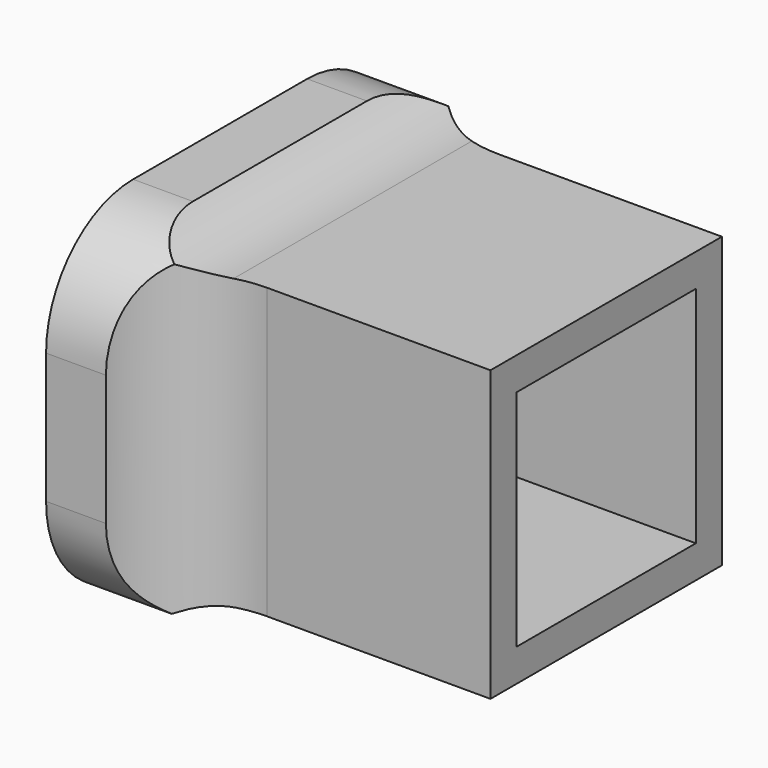
from build123d import *

# Parameters (mm, degrees)
F0_W         = 2.75
F0_H         = 20
F1_DEPTH     = 16
F2_W         = 5.15
F2_H         = 10.3
F3_DEPTH     = 2.75
F4_DEPTH     = 15
F5_T1_DEPTH  = 13.2999992773
F5_T3_DEPTH  = 13.2999992773
F5_T9_DEPTH  = 21.6634917276
F5_T14_DEPTH = 25.0997612432
F5_T22_DEPTH = 21.6634917276
F5_T27_DEPTH = 25.0997612432
F5_T35_DEPTH = 22.0158699277
F5_T40_DEPTH = 25.0997612432
F5_T48_DEPTH = 25.0997612432
F5_T53_DEPTH = 22.0158699277
F6_R         = 5


# Not quite as in the source:
# - a fillet or chamfer that OpenCascade refuses, or shapes differently, is made with other operations: its cross-section is extruded or revolved along the edge and cut away or added
# - a feature names something its author has since deleted; it is built from what else it names


with BuildPart() as f1:
    # F0 (on Top) → F1 (new body)
    with BuildSketch(Plane.XY):
        Rectangle(F0_W, F0_H)
    extrude(amount=F1_DEPTH)

    # F2 (on face) → F3 (join)
    with BuildSketch(Plane.YZ.offset(1.375)):
        Polygon((0, 16), (-10, 16), (-10, 0), (0, 0), (0, 1.4159553841), (-6.6499996386, 1.4159553841), (-6.6499996386, 14.7159546614), (0, 14.7159546614), align=None)
        Polygon((10, 16), (0, 16), (0, 14.7159546614), (6.6499996386, 14.7159546614), (6.6499996386, 1.4159553841), (0, 1.4159553841), (0, 0), (10, 0), align=None)
        with Locations((-2.575, 8.0659550227)):
            Rectangle(F2_W, F2_H)
        with Locations((2.575, 8.0659550227)):
            Rectangle(F2_W, F2_H)
        Polygon((0, 13.2159550227), (0, 14.7159546614), (-6.6499996386, 14.7159546614), (-6.6499996386, 1.4159553841), (0, 1.4159553841), (0, 2.9159550227), (-5.15, 2.9159550227), (-5.15, 13.2159550227), align=None)
        Polygon((6.6499996386, 14.7159546614), (0, 14.7159546614), (0, 13.2159550227), (5.15, 13.2159550227), (5.15, 2.9159550227), (0, 2.9159550227), (0, 1.4159553841), (6.6499996386, 1.4159553841), align=None)
    extrude(amount=-F3_DEPTH)

    # F2 (on face) → F4 (join)
    with BuildSketch(Plane.YZ.offset(1.375)):
        Polygon((0, 13.2159550227), (0, 14.7159546614), (-6.6499996386, 14.7159546614), (-6.6499996386, 1.4159553841), (0, 1.4159553841), (0, 2.9159550227), (-5.15, 2.9159550227), (-5.15, 13.2159550227), align=None)
        Polygon((6.6499996386, 14.7159546614), (0, 14.7159546614), (0, 13.2159550227), (5.15, 13.2159550227), (5.15, 2.9159550227), (0, 2.9159550227), (0, 1.4159553841), (6.6499996386, 1.4159553841), align=None)
    extrude(amount=F4_DEPTH)

    # F5: fillet of radius 5 on 6 edges, made by hand

    # F5_s2 → F5_t1 (join)
    with BuildSketch(Plane.XZ.offset(-6.6499996386)):
        with BuildLine():
            ThreePointArc((1.375, 16), (2.9287180617, 15.0479907955), (4.7203969801, 14.7159546614))
            Line((4.7203969801, 14.7159546614), (1.375, 14.7159546614))
            Line((1.375, 14.7159546614), (1.375, 16))
        make_face()
        with BuildLine():
            ThreePointArc((1.375, 0), (2.9798891295, 1.0484613517), (4.8613482602, 1.4159553841))
            Line((4.8613482602, 1.4159553841), (1.375, 1.4159553841))
            Line((1.375, 1.4159553841), (1.375, 0))
        make_face()
    extrude(amount=F5_T1_DEPTH)

    # F5_s4 → F5_t3 (join)
    with BuildSketch(Plane.XY.offset(1.4159553841)):
        with BuildLine():
            ThreePointArc((1.375, -10), (3.2009454046, -7.5726231419), (6.0949047864, -6.6499996386))
            Line((6.0949047864, -6.6499996386), (1.375, -6.6499996386))
            Line((1.375, -6.6499996386), (1.375, -10))
        make_face()
        with BuildLine():
            ThreePointArc((1.375, 10), (3.2009454046, 7.5726231419), (6.0949047864, 6.6499996386))
            Line((6.0949047864, 6.6499996386), (1.375, 6.6499996386))
            Line((1.375, 6.6499996386), (1.375, 10))
        make_face()
    extrude(amount=F5_T3_DEPTH)


with BuildPart() as f5_tool7:
    # F5_s8 → F5_t9 (new body)
    with BuildSketch(Plane.XZ.offset(-15.013492089)):
        with BuildLine():
            ThreePointArc((1.375, 16), (2.9287180617, 15.0479907955), (4.7203969801, 14.7159546614))
            Line((4.7203969801, 14.7159546614), (1.375, 14.7159546614))
            Line((1.375, 14.7159546614), (1.375, 16))
        make_face()
    extrude(amount=F5_T9_DEPTH)

    split(bisect_by=Plane.XZ.offset(-10), keep=Keep.TOP)

    split(bisect_by=Plane.XZ.offset(-6.6499996386), keep=Keep.BOTTOM)


with BuildPart() as f5_tool12:
    # F5_s13 → F5_t14 (new body)
    with BuildSketch(Plane.XY.offset(1.4159553841)):
        with BuildLine():
            ThreePointArc((1.375, 10), (3.2009454046, 7.5726231419), (6.0949047864, 6.6499996386))
            Line((6.0949047864, 6.6499996386), (1.375, 6.6499996386))
            Line((1.375, 6.6499996386), (1.375, 10))
        make_face()
    extrude(amount=F5_T14_DEPTH)

    split(bisect_by=Plane.XY.offset(16), keep=Keep.BOTTOM)

    split(bisect_by=Plane.XY.offset(14.7159546614), keep=Keep.TOP)


with BuildPart() as f5_tool7_1:
    add(f5_tool7.part)

    # F5_t17: intersect F5_tool12
    add(f5_tool12.part, mode=Mode.INTERSECT)


with BuildPart() as f1_1:
    add(f1.part)

    # F5_t5: union F5_tool7
    add(f5_tool7_1.part)


with BuildPart() as f5_tool20:
    # F5_s21 → F5_t22 (new body)
    with BuildSketch(Plane.XZ.offset(-6.6499996386)):
        with BuildLine():
            ThreePointArc((1.375, 16), (2.9287180617, 15.0479907955), (4.7203969801, 14.7159546614))
            Line((4.7203969801, 14.7159546614), (1.375, 14.7159546614))
            Line((1.375, 14.7159546614), (1.375, 16))
        make_face()
    extrude(amount=F5_T22_DEPTH)

    split(bisect_by=Plane.XZ.offset(10), keep=Keep.BOTTOM)

    split(bisect_by=Plane.XZ.offset(6.6499996386), keep=Keep.TOP)


with BuildPart() as f5_tool25:
    # F5_s26 → F5_t27 (new body)
    with BuildSketch(Plane.XY.offset(26.5157166273)):
        with BuildLine():
            ThreePointArc((1.375, -10), (3.2009454046, -7.5726231419), (6.0949047864, -6.6499996386))
            Line((6.0949047864, -6.6499996386), (1.375, -6.6499996386))
            Line((1.375, -6.6499996386), (1.375, -10))
        make_face()
    extrude(amount=-F5_T27_DEPTH)

    split(bisect_by=Plane.XY.offset(16), keep=Keep.BOTTOM)

    split(bisect_by=Plane.XY.offset(14.7159546614), keep=Keep.TOP)


with BuildPart() as f5_tool20_1:
    add(f5_tool20.part)

    # F5_t30: intersect F5_tool25
    add(f5_tool25.part, mode=Mode.INTERSECT)


with BuildPart() as f1_2:
    add(f1_1.part)

    # F5_t18: union F5_tool20
    add(f5_tool20_1.part)


with BuildPart() as f5_tool33:
    # F5_s34 → F5_t35 (new body)
    with BuildSketch(Plane.XZ.offset(15.365870289)):
        with BuildLine():
            ThreePointArc((1.375, 0), (2.9798891295, 1.0484613517), (4.8613482602, 1.4159553841))
            Line((4.8613482602, 1.4159553841), (1.375, 1.4159553841))
            Line((1.375, 1.4159553841), (1.375, 0))
        make_face()
    extrude(amount=-F5_T35_DEPTH)

    split(bisect_by=Plane.XZ.offset(10), keep=Keep.BOTTOM)

    split(bisect_by=Plane.XZ.offset(6.6499996386), keep=Keep.TOP)


with BuildPart() as f5_tool38:
    # F5_s39 → F5_t40 (new body)
    with BuildSketch(Plane.XY.offset(14.7159546614)):
        with BuildLine():
            ThreePointArc((1.375, -10), (3.2009454046, -7.5726231419), (6.0949047864, -6.6499996386))
            Line((6.0949047864, -6.6499996386), (1.375, -6.6499996386))
            Line((1.375, -6.6499996386), (1.375, -10))
        make_face()
    extrude(amount=-F5_T40_DEPTH)

    split(bisect_by=Plane.XY, keep=Keep.TOP)

    split(bisect_by=Plane.XY.offset(1.4159553841), keep=Keep.BOTTOM)


with BuildPart() as f5_tool33_1:
    add(f5_tool33.part)

    # F5_t43: intersect F5_tool38
    add(f5_tool38.part, mode=Mode.INTERSECT)


with BuildPart() as f1_3:
    add(f1_2.part)

    # F5_t31: union F5_tool33
    add(f5_tool33_1.part)


with BuildPart() as f5_tool46:
    # F5_s47 → F5_t48 (new body)
    with BuildSketch(Plane.XY.offset(-10.3838065819)):
        with BuildLine():
            ThreePointArc((1.375, 10), (3.2009454046, 7.5726231419), (6.0949047864, 6.6499996386))
            Line((6.0949047864, 6.6499996386), (1.375, 6.6499996386))
            Line((1.375, 6.6499996386), (1.375, 10))
        make_face()
    extrude(amount=F5_T48_DEPTH)

    split(bisect_by=Plane.XY, keep=Keep.TOP)

    split(bisect_by=Plane.XY.offset(1.4159553841), keep=Keep.BOTTOM)


with BuildPart() as f5_tool51:
    # F5_s52 → F5_t53 (new body)
    with BuildSketch(Plane.XZ.offset(6.6499996386)):
        with BuildLine():
            ThreePointArc((1.375, 0), (2.9798891295, 1.0484613517), (4.8613482602, 1.4159553841))
            Line((4.8613482602, 1.4159553841), (1.375, 1.4159553841))
            Line((1.375, 1.4159553841), (1.375, 0))
        make_face()
    extrude(amount=-F5_T53_DEPTH)

    split(bisect_by=Plane.XZ.offset(-10), keep=Keep.TOP)

    split(bisect_by=Plane.XZ.offset(-6.6499996386), keep=Keep.BOTTOM)


with BuildPart() as f5_tool46_1:
    add(f5_tool46.part)

    # F5_t56: intersect F5_tool51
    add(f5_tool51.part, mode=Mode.INTERSECT)


with BuildPart() as f1_4:
    add(f1_3.part)

    # F5_t44: union F5_tool46
    add(f5_tool46_1.part)

    # F6
    f6_edges = [f1_4.edges().sort_by_distance(p)[0] for p in [
        (0, -10, 0),
        (0, -10, 16),
        (0, 10, 16),
        (0, 10, 0),
    ]]
    fillet(f6_edges, radius=F6_R)


solid = f1_4.part
